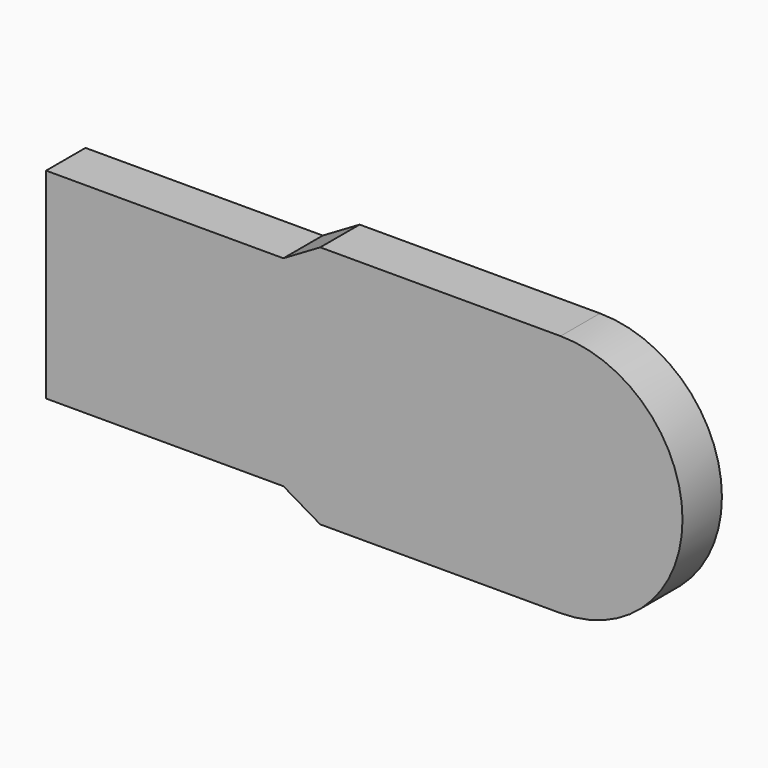
from build123d import *

# Parameters (mm, degrees)
F0_W     = 15.24
F0_H     = 15.4686
F1_DEPTH = 3.1242


# Not quite as in the source:
# - the program builds the solid bodies; features that only make, move or delete a surface that nothing else refers to are left out


with BuildPart() as f1:
    # F0 (on Front) → F1 (new body)
    with BuildSketch(Plane.XZ):
        Polygon((-7.62, -7.7343), (-7.62, 7.7343), (-9.9592747303, 6.3627), (-20.8109102848, 0), (-9.9592747303, -6.3627), align=None)
        Rectangle(F0_W, F0_H)
        with BuildLine():
            ThreePointArc((7.62, -7.7343), (15.3543, 0), (7.62, 7.7343))
            Line((7.62, 7.7343), (7.62, -7.7343))
        make_face()
        Polygon((-20.8109102848, 0), (-9.9592747303, 6.3627), (-22.6592747303, 6.3627), (-25.0076241791, 6.3627), (-25.0076241791, -6.3627), (-22.6592747303, -6.3627), (-9.9592747303, -6.3627), align=None)
    extrude(amount=F1_DEPTH)


solid = f1.part
